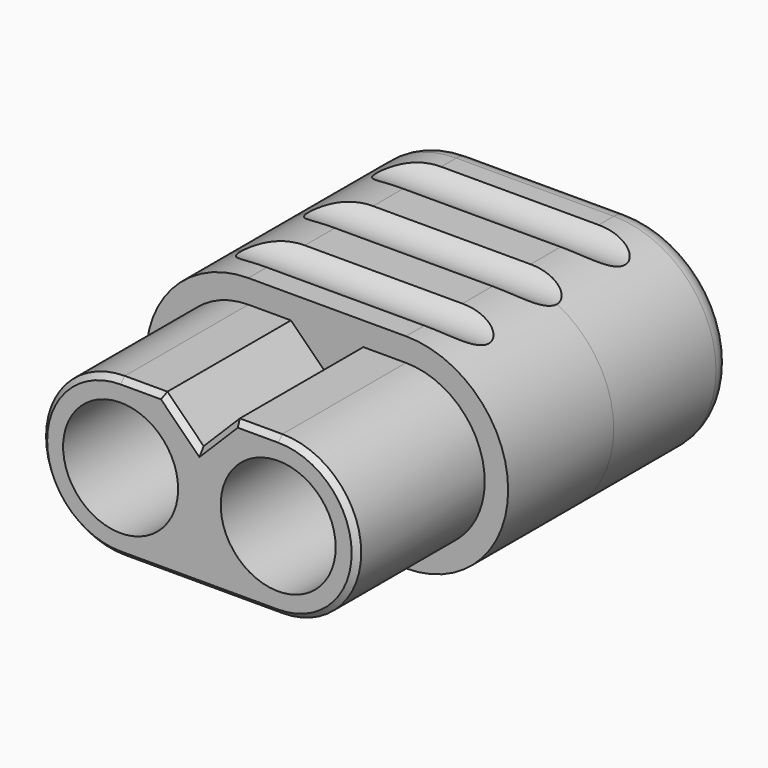
from build123d import *

# Parameters (mm, degrees)
F0_R      = 2.8
F1_DEPTH  = 1.5
F0_R_2    = 2.425
F2_DEPTH  = 2.2
F3_R      = 2.7
F4_DEPTH  = 2.5
F5_R      = 2.7
F6_DEPTH  = 7.5
F7_R      = 3.2
F8_DEPTH  = 7
F9_R      = 1
F10_SIZE  = 0.25
F11_R     = 1.5
F12_DEPTH = 8.5


# Not quite as in the source:
# - a feature names something its author has since deleted; it is built from what else it names


with BuildPart() as f1:
    # F0 (on Front) → F1 (new body)
    with BuildSketch(Plane.XZ):
        with BuildLine():
            Line((0, 4.8), (-3.7, 4.8))
            ThreePointArc((-3.7, 4.8), (-7.0941125497, 3.3941125497), (-8.5, 0))
            ThreePointArc((-8.5, 0), (-7.0941125497, -3.3941125497), (-3.7, -4.8))
            Line((-3.7, -4.8), (0, -4.8))
            Line((0, -4.8), (3.7, -4.8))
            ThreePointArc((3.7, -4.8), (7.0941125497, -3.3941125497), (8.5, 0))
            ThreePointArc((8.5, 0), (7.0941125497, 3.3941125497), (3.7, 4.8))
            Line((3.7, 4.8), (0, 4.8))
        make_face()
        with Locations((-3.7, 0)):
            Circle(F0_R, mode=Mode.SUBTRACT)
        with Locations((3.7, 0)):
            Circle(F0_R, mode=Mode.SUBTRACT)
    extrude(amount=-F1_DEPTH)

    # F0 (on Front) → F2 (join)
    with BuildSketch(Plane.XZ):
        with BuildLine():
            Line((0, 4.8), (-3.7, 4.8))
            ThreePointArc((-3.7, 4.8), (-7.0941125497, 3.3941125497), (-8.5, 0))
            ThreePointArc((-8.5, 0), (-7.0941125497, -3.3941125497), (-3.7, -4.8))
            Line((-3.7, -4.8), (0, -4.8))
            Line((0, -4.8), (3.7, -4.8))
            ThreePointArc((3.7, -4.8), (7.0941125497, -3.3941125497), (8.5, 0))
            ThreePointArc((8.5, 0), (7.0941125497, 3.3941125497), (3.7, 4.8))
            Line((3.7, 4.8), (0, 4.8))
        make_face()
        with Locations((-3.7, 0)):
            Circle(F0_R, mode=Mode.SUBTRACT)
        with Locations((3.7, 0)):
            Circle(F0_R, mode=Mode.SUBTRACT)
        with Locations((-3.7, 0)):
            Circle(F0_R)
        with Locations((-3.7, 0)):
            Circle(F0_R_2, mode=Mode.SUBTRACT)
        with Locations((3.7, 0)):
            Circle(F0_R)
        with Locations((3.7, 0)):
            Circle(F0_R_2, mode=Mode.SUBTRACT)
    extrude(amount=F2_DEPTH)

    # F3 (on face) → F4 (join)
    with BuildSketch(Plane.XZ.offset(2.2)):
        with BuildLine():
            ThreePointArc((3.7, -4.8), (8.5, 0), (3.7, 4.8))
            Line((3.7, 4.8), (-3.7, 4.8))
            ThreePointArc((-3.7, 4.8), (-8.5, 0), (-3.7, -4.8))
            Line((-3.7, -4.8), (3.7, -4.8))
        make_face()
        with Locations((-3.7, 0)):
            Circle(F3_R, mode=Mode.SUBTRACT)
        with Locations((3.7, 0)):
            Circle(F3_R, mode=Mode.SUBTRACT)
    extrude(amount=F4_DEPTH)

    # F5 (on face) → F6 (join)
    with BuildSketch(Plane.XZ.offset(4.7)):
        with BuildLine():
            ThreePointArc((-3.7, 3.7), (-7.4, 0), (-3.7, -3.7))
            Line((-3.7, -3.7), (0, -3.7))
            Line((0, -3.7), (3.7, -3.7))
            ThreePointArc((3.7, -3.7), (7.4, 0), (3.7, 3.7))
            Line((3.7, 3.7), (1.7, 3.7))
            Line((1.7, 3.7), (0, 2))
            Line((0, 2), (-1.7, 3.7))
            Line((-1.7, 3.7), (-3.7, 3.7))
        make_face()
        with Locations((-3.7, 0)):
            Circle(F5_R, mode=Mode.SUBTRACT)
        with Locations((3.7, 0)):
            Circle(F5_R, mode=Mode.SUBTRACT)
    extrude(amount=F6_DEPTH)

    # F7 (on face) → F8 (join)
    with BuildSketch(Plane(origin=(0, 1.5, 0), x_dir=(-1, 0, 0), z_dir=(0, 1, 0))):
        with BuildLine():
            ThreePointArc((3.7, -4.8), (8.5, 0), (3.7, 4.8))
            Line((3.7, 4.8), (-3.7, 4.8))
            ThreePointArc((-3.7, 4.8), (-8.5, 0), (-3.7, -4.8))
            Line((-3.7, -4.8), (3.7, -4.8))
        make_face()
        with Locations((-3.7, 0)):
            Circle(F7_R, mode=Mode.SUBTRACT)
        with Locations((3.7, 0)):
            Circle(F7_R, mode=Mode.SUBTRACT)
    extrude(amount=F8_DEPTH)

    # F9
    f9_edges = [f1.edges().sort_by_distance(p)[0] for p in [
        (0, 8.5, 4.8),
    ]]
    fillet(f9_edges, radius=F9_R)

    # F10
    f10_edges = [f1.edges().sort_by_distance(p)[0] for p in [
        (-2.7, -12.2, 3.7),
        (-0.85, -12.2, 2.85),
        (0.85, -12.2, 2.85),
    ]]
    chamfer(f10_edges, length=F10_SIZE)

    # F11 (on Right) → F12 (cut, symmetric)
    with BuildSketch(Plane.YZ):
        with Locations((1.5, 5.8)):
            Circle(F11_R)
        with Locations((-2.5, 5.8)):
            Circle(F11_R)
        with Locations((-2.5, -5.8)):
            Circle(F11_R)
        with Locations((1.5, -5.8)):
            Circle(F11_R)
        with Locations((5.5, -5.8)):
            Circle(F11_R)
        with Locations((5.5, 5.8)):
            Circle(F11_R)
    extrude(amount=F12_DEPTH, both=True, mode=Mode.SUBTRACT)


solid = f1.part
